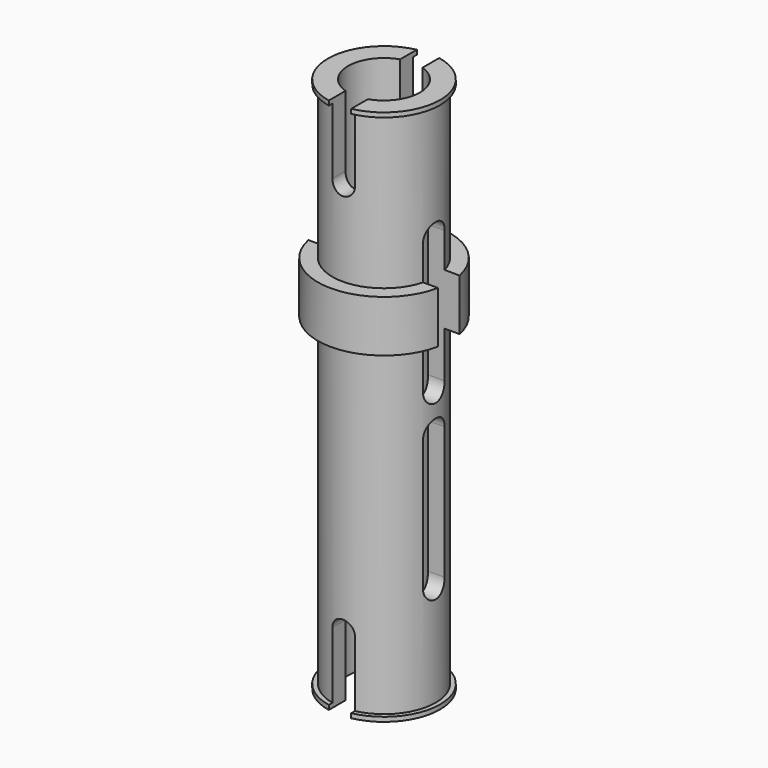
from build123d import *

# Parameters (mm, degrees)
F0_R      = 2.95
F1_DEPTH  = 11.95
F2_R      = 2.95
F2_R_2    = 2.3
F3_DEPTH  = 7
F4_R      = 2.95
F4_R_2    = 2.3
F5_DEPTH  = 14.6
F6_R      = 1.6
F7_DEPTH  = 23.901
F9_DEPTH  = 12.5
F10_W     = 0.2
F10_H     = 0.2
F12_DEPTH = 12.5
F13_DEPTH = 12.5
F15_DEPTH = 12.5


# Not quite as in the source:
# - a pattern or mirror of a feature is missing from the dataset's text; its kind, count and spacing are read off the source's solid


with BuildPart() as f1:
    # F0 (on Top) → F1 (new body, symmetric)
    with BuildSketch(Plane.XY):
        Circle(F0_R)
    extrude(amount=F1_DEPTH, both=True)

    # F2 (on face) → F3 (cut)
    with BuildSketch(Plane.XY.offset(11.95)):
        Circle(F2_R)
        Circle(F2_R_2, mode=Mode.SUBTRACT)
    extrude(amount=-F3_DEPTH, mode=Mode.SUBTRACT)

    # F4 (on face) → F5 (cut)
    with BuildSketch(Plane(origin=(0, 0, -11.95), x_dir=(1, 0, 0), z_dir=(0, 0, -1))):
        Circle(F4_R)
        Circle(F4_R_2, mode=Mode.SUBTRACT)
    extrude(amount=-F5_DEPTH, mode=Mode.SUBTRACT)

    # F6 (on face) → F7 (cut, through all)
    with BuildSketch(Plane.XY.offset(11.95)):
        Circle(F6_R)
    extrude(amount=-F7_DEPTH, mode=Mode.SUBTRACT)

    # F8 (on Front) → F9 (cut, symmetric)
    with BuildSketch(Plane.XZ):
        with BuildLine():
            ThreePointArc((0.5, 8.8), (0, 9.3), (-0.5, 8.8))
            Line((-0.5, 8.8), (0.5, 8.8))
        make_face()
        with BuildLine():
            Line((-0.5, 11.95), (-0.5, 8.8))
            ThreePointArc((-0.5, 8.8), (0, 9.3), (0.5, 8.8))
            Line((0.5, 8.8), (0.5, 11.95))
            Line((0.5, 11.95), (-0.5, 11.95))
        make_face()
        with BuildLine():
            Line((0.5, 8.8), (-0.5, 8.8))
            ThreePointArc((-0.5, 8.8), (0, 8.3), (0.5, 8.8))
        make_face()
        with BuildLine():
            Line((-0.5, -8.8), (-0.5, -11.95))
            Line((-0.5, -11.95), (0.5, -11.95))
            Line((0.5, -11.95), (0.5, -8.8))
            ThreePointArc((0.5, -8.8), (0, -9.3), (-0.5, -8.8))
        make_face()
        with BuildLine():
            ThreePointArc((0.5, -8.8), (0, -8.3), (-0.5, -8.8))
            Line((-0.5, -8.8), (0.5, -8.8))
        make_face()
        with BuildLine():
            Line((0.5, -8.8), (-0.5, -8.8))
            ThreePointArc((-0.5, -8.8), (0, -9.3), (0.5, -8.8))
        make_face()
    extrude(amount=F9_DEPTH, both=True, mode=Mode.SUBTRACT)

    # F10 (on Front) → F11 (revolve)
    with BuildSketch(Plane.XZ):
        with Locations((2.4, 11.85)):
            Rectangle(F10_W, F10_H)
    f11 = revolve(axis=Axis((0, 0, 11.95), (0, 0, 1)))

    # F11_copies: F11 across plane
    add(f11.mirror(Plane(origin=(0, 0, 0), x_dir=(-1, 0, 0), z_dir=(0, 0, -1))))

    # F8 (on Front) → F12 (cut, symmetric)
    with BuildSketch(Plane.XZ):
        with BuildLine():
            ThreePointArc((0.5, 8.8), (0, 9.3), (-0.5, 8.8))
            Line((-0.5, 8.8), (0.5, 8.8))
        make_face()
        with BuildLine():
            Line((-0.5, 11.95), (-0.5, 8.8))
            ThreePointArc((-0.5, 8.8), (0, 9.3), (0.5, 8.8))
            Line((0.5, 8.8), (0.5, 11.95))
            Line((0.5, 11.95), (-0.5, 11.95))
        make_face()
        with BuildLine():
            Line((0.5, 8.8), (-0.5, 8.8))
            ThreePointArc((-0.5, 8.8), (0, 8.3), (0.5, 8.8))
        make_face()
        with BuildLine():
            Line((-0.5, -8.8), (-0.5, -11.95))
            Line((-0.5, -11.95), (0.5, -11.95))
            Line((0.5, -11.95), (0.5, -8.8))
            ThreePointArc((0.5, -8.8), (0, -9.3), (-0.5, -8.8))
        make_face()
        with BuildLine():
            ThreePointArc((0.5, -8.8), (0, -8.3), (-0.5, -8.8))
            Line((-0.5, -8.8), (0.5, -8.8))
        make_face()
        with BuildLine():
            Line((0.5, -8.8), (-0.5, -8.8))
            ThreePointArc((-0.5, -8.8), (0, -9.3), (0.5, -8.8))
        make_face()
    extrude(amount=F12_DEPTH, both=True, mode=Mode.SUBTRACT)

    # F8 (on Front) → F13 (cut, symmetric)
    with BuildSketch(Plane.XZ):
        with BuildLine():
            ThreePointArc((0.5, 8.8), (0, 9.3), (-0.5, 8.8))
            Line((-0.5, 8.8), (0.5, 8.8))
        make_face()
        with BuildLine():
            Line((-0.5, 11.95), (-0.5, 8.8))
            ThreePointArc((-0.5, 8.8), (0, 9.3), (0.5, 8.8))
            Line((0.5, 8.8), (0.5, 11.95))
            Line((0.5, 11.95), (-0.5, 11.95))
        make_face()
        with BuildLine():
            Line((0.5, 8.8), (-0.5, 8.8))
            ThreePointArc((-0.5, 8.8), (0, 8.3), (0.5, 8.8))
        make_face()
        with BuildLine():
            Line((-0.5, -8.8), (-0.5, -11.95))
            Line((-0.5, -11.95), (0.5, -11.95))
            Line((0.5, -11.95), (0.5, -8.8))
            ThreePointArc((0.5, -8.8), (0, -9.3), (-0.5, -8.8))
        make_face()
        with BuildLine():
            ThreePointArc((0.5, -8.8), (0, -8.3), (-0.5, -8.8))
            Line((-0.5, -8.8), (0.5, -8.8))
        make_face()
        with BuildLine():
            Line((0.5, -8.8), (-0.5, -8.8))
            ThreePointArc((-0.5, -8.8), (0, -9.3), (0.5, -8.8))
        make_face()
    extrude(amount=F13_DEPTH, both=True, mode=Mode.SUBTRACT)

    # F14 (on Right) → F15 (cut, symmetric)
    with BuildSketch(Plane.YZ):
        with BuildLine():
            ThreePointArc((-0.6, 0.6), (0, 0), (0.6, 0.6))
            Line((0.6, 0.6), (-0.6, 0.6))
        make_face()
        with BuildLine():
            ThreePointArc((-0.6, 0.6), (0, 1.2), (0.6, 0.6))
            Line((0.6, 0.6), (0.6, 6.5))
            ThreePointArc((0.6, 6.5), (0, 5.9), (-0.6, 6.5))
            Line((-0.6, 6.5), (-0.6, 0.6))
        make_face()
        with BuildLine():
            Line((-0.6, 0.6), (0.6, 0.6))
            ThreePointArc((0.6, 0.6), (0, 1.2), (-0.6, 0.6))
        make_face()
        with BuildLine():
            ThreePointArc((-0.6, 6.5), (0, 5.9), (0.6, 6.5))
            Line((0.6, 6.5), (-0.6, 6.5))
        make_face()
        with BuildLine():
            Line((-0.6, 6.5), (0.6, 6.5))
            ThreePointArc((0.6, 6.5), (0, 7.1), (-0.6, 6.5))
        make_face()
        with BuildLine():
            ThreePointArc((-0.6, -7.1), (0, -7.7), (0.6, -7.1))
            Line((0.6, -7.1), (-0.6, -7.1))
        make_face()
        with BuildLine():
            ThreePointArc((-0.6, -7.1), (0, -6.5), (0.6, -7.1))
            Line((0.6, -7.1), (0.6, -1.2))
            ThreePointArc((0.6, -1.2), (0, -1.8), (-0.6, -1.2))
            Line((-0.6, -1.2), (-0.6, -7.1))
        make_face()
        with BuildLine():
            Line((-0.6, -7.1), (0.6, -7.1))
            ThreePointArc((0.6, -7.1), (0, -6.5), (-0.6, -7.1))
        make_face()
        with BuildLine():
            ThreePointArc((-0.6, -1.2), (0, -1.8), (0.6, -1.2))
            Line((0.6, -1.2), (-0.6, -1.2))
        make_face()
        with BuildLine():
            Line((-0.6, -1.2), (0.6, -1.2))
            ThreePointArc((0.6, -1.2), (0, -0.6), (-0.6, -1.2))
        make_face()
    extrude(amount=F15_DEPTH, both=True, mode=Mode.SUBTRACT)


solid = f1.part
